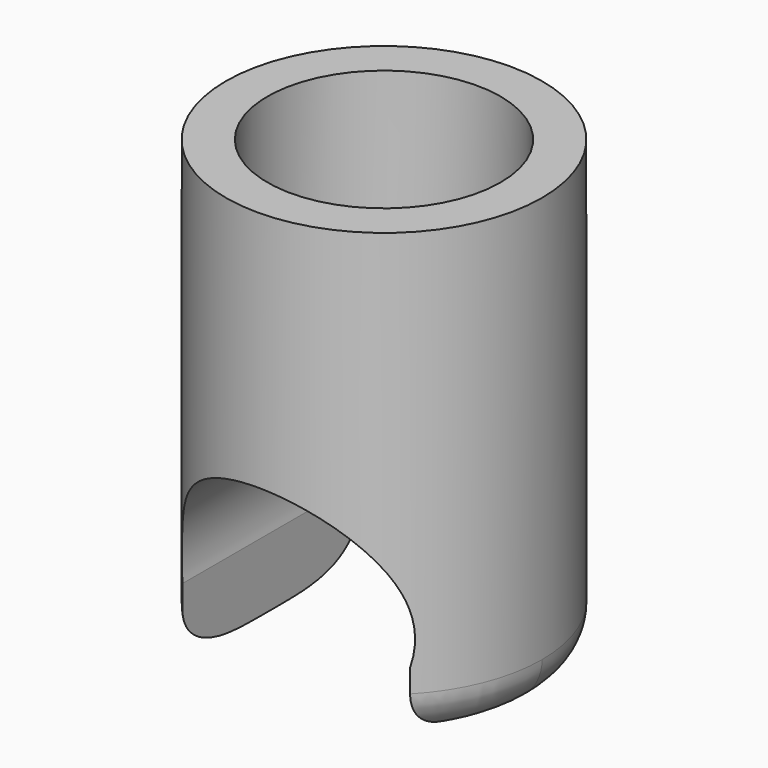
from build123d import *

# Parameters (mm, degrees)
F0_R        = 11.1125
F0_R_2      = 8.1915
F1_DEPTH    = 12.7
F2_R        = 11.1125
F3_DEPTH    = 19.05
F5_DEPTH    = 19.05
F6_T2_ANGLE = 169.7302536888
F6_T4_ANGLE = 84.8533787692
F6_T6_ANGLE = 84.8533787692


# Not quite as in the source:
# - a fillet or chamfer that OpenCascade refuses, or shapes differently, is made with other operations: its cross-section is extruded or revolved along the edge and cut away or added


with BuildPart() as f1:
    # F0 (on Top) → F1 (new body)
    with BuildSketch(Plane.XY):
        Circle(F0_R)
        Circle(F0_R_2, mode=Mode.SUBTRACT)
    extrude(amount=F1_DEPTH)

    # F2 (on Top) → F3 (join)
    with BuildSketch(Plane.XY):
        Circle(F2_R)
    extrude(amount=-F3_DEPTH)

    # F4 (on Front) → F5 (cut, symmetric)
    with BuildSketch(Plane.XZ):
        with BuildLine():
            Line((8.0039083969, -20.9773854417), (8.0039083969, -14.2491279898))
            ThreePointArc((8.0039083969, -14.2491279898), (6.3788176707, -7.3669087446), (0, -4.3146068702))
            ThreePointArc((0, -4.3146068702), (-6.3788176707, -7.3669087446), (-8.0039083969, -14.2491279898))
            Line((-8.0039083969, -14.2491279898), (-8.0039083969, -20.9773854417))
            Line((-8.0039083969, -20.9773854417), (8.0039083969, -20.9773854417))
        make_face()
    extrude(amount=F5_DEPTH, both=True, mode=Mode.SUBTRACT)

    # F6: fillet of radius 3.175 on 3 edges, made by hand

    # F6_s1 → F6_t2 (revolve, cut)
    with BuildSketch(Plane(origin=(0, 0, 0), x_dir=(0, 0, 1), z_dir=(0.9959867753, 0.0895005221, 0))):
        with BuildLine():
            ThreePointArc((-15.875, -11.1125), (-18.1200640303, -10.1825640303), (-19.05, -7.9375))
            Line((-19.05, -7.9375), (-19.05, -11.1125))
            Line((-19.05, -11.1125), (-15.875, -11.1125))
        make_face()
    revolve(axis=Axis((0, 0, -19.05), (0, 0, 1)), revolution_arc=F6_T2_ANGLE, mode=Mode.SUBTRACT)

    # F6_s3 → F6_t4 (revolve, cut)
    with BuildSketch(Plane(origin=(0, 0, 0), x_dir=(0, 0, 1), z_dir=(-0.9959684029, -0.08970474, 0))):
        with BuildLine():
            ThreePointArc((-15.875, -11.1125), (-18.1200640303, -10.1825640303), (-19.05, -7.9375))
            Line((-19.05, -7.9375), (-19.05, -11.1125))
            Line((-19.05, -11.1125), (-15.875, -11.1125))
        make_face()
    revolve(axis=Axis((0, 0, -19.05), (0, 0, 1)), revolution_arc=F6_T4_ANGLE, mode=Mode.SUBTRACT)

    # F6_s5 → F6_t6 (revolve, cut)
    with BuildSketch(Plane.XZ):
        with BuildLine():
            ThreePointArc((11.1125, -15.875), (10.1825640303, -18.1200640303), (7.9375, -19.05))
            Line((7.9375, -19.05), (11.1125, -19.05))
            Line((11.1125, -19.05), (11.1125, -15.875))
        make_face()
    revolve(axis=Axis((0, 0, -19.05), (0, 0, 1)), revolution_arc=F6_T6_ANGLE, mode=Mode.SUBTRACT)


solid = f1.part
